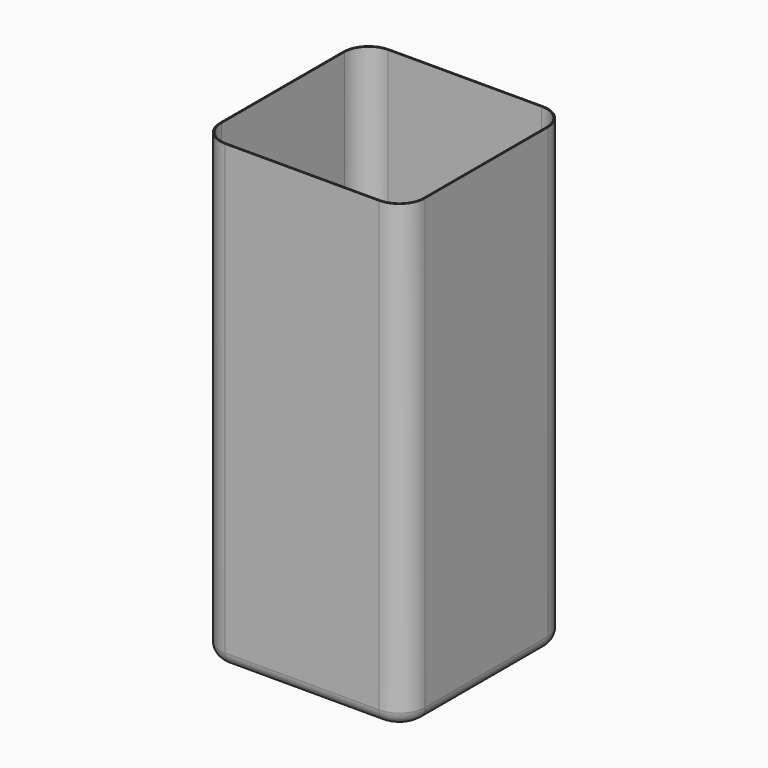
from build123d import *

# Parameters (mm, degrees)
F1_DEPTH     = 914.4
F2_R         = 25.4
F3_T1_DEPTH  = 1041.4
F3_T4_ANGLE  = 90
F3_T6_ANGLE  = 90
F3_T8_ANGLE  = 90
F3_T10_ANGLE = 90
F4_T         = -2.54


# Not quite as in the source:
# - a fillet or chamfer that OpenCascade refuses, or shapes differently, is made with other operations: its cross-section is extruded or revolved along the edge and cut away or added


with BuildPart() as f1:
    # F0 (on Top) → F1 (new body)
    with BuildSketch(Plane.XY):
        Polygon((203.2, -203.2), (203.2, 0), (203.2, 203.2), (-203.2, 203.2), (-203.2, -203.2), align=None)
    extrude(amount=F1_DEPTH)

    # F2
    f2_edges = [f1.edges().sort_by_distance(p)[0] for p in [
        (-203.2, 0, 0),
        (0, 203.2, 0),
        (0, -203.2, 0),
        (203.2, 0, 0),
    ]]
    fillet(f2_edges, radius=F2_R)

    # F3: fillet of radius 50.8 on 4 edges, made by hand

    # F3_s2 → F3_t1 (cut)
    with BuildSketch(Plane.XY):
        with BuildLine():
            ThreePointArc((-152.4, 203.2), (-188.3210244843, 188.3210244843), (-203.2, 152.4))
            Line((-203.2, 152.4), (-203.2, 203.2))
            Line((-203.2, 203.2), (-152.4, 203.2))
        make_face()
        with BuildLine():
            ThreePointArc((-152.4, -203.2), (-188.3210244843, -188.3210244843), (-203.2, -152.4))
            Line((-203.2, -152.4), (-203.2, -203.2))
            Line((-203.2, -203.2), (-152.4, -203.2))
        make_face()
        with BuildLine():
            ThreePointArc((203.2, 152.4), (188.3210244843, 188.3210244843), (152.4, 203.2))
            Line((152.4, 203.2), (203.2, 203.2))
            Line((203.2, 203.2), (203.2, 152.4))
        make_face()
        with BuildLine():
            ThreePointArc((203.2, -152.4), (188.3210244843, -188.3210244843), (152.4, -203.2))
            Line((152.4, -203.2), (203.2, -203.2))
            Line((203.2, -203.2), (203.2, -152.4))
        make_face()
    extrude(amount=F3_T1_DEPTH, mode=Mode.SUBTRACT)

    # F3_s3 → F3_t4 (revolve, cut)
    with BuildSketch(Plane.XZ.offset(152.4)):
        with BuildLine():
            ThreePointArc((177.8, 0), (195.7605122421, 7.4394877579), (203.2, 25.4))
            Line((203.2, 25.4), (203.2, 0))
            Line((203.2, 0), (177.8, 0))
        make_face()
    revolve(axis=Axis((152.4, -152.4, 0), (0, 0, -1)), revolution_arc=F3_T4_ANGLE, mode=Mode.SUBTRACT)

    # F3_s5 → F3_t6 (revolve, cut)
    with BuildSketch(Plane.YZ.offset(152.4)):
        with BuildLine():
            ThreePointArc((177.8, 0), (195.7605122421, 7.4394877579), (203.2, 25.4))
            Line((203.2, 25.4), (203.2, 0))
            Line((203.2, 0), (177.8, 0))
        make_face()
    revolve(axis=Axis((152.4, 152.4, 0), (0, 0, -1)), revolution_arc=F3_T6_ANGLE, mode=Mode.SUBTRACT)

    # F3_s7 → F3_t8 (revolve, cut)
    with BuildSketch(Plane.YZ.offset(-152.4)):
        with BuildLine():
            ThreePointArc((-177.8, 0), (-195.7605122421, 7.4394877579), (-203.2, 25.4))
            Line((-203.2, 25.4), (-203.2, 0))
            Line((-203.2, 0), (-177.8, 0))
        make_face()
    revolve(axis=Axis((-152.4, -152.4, 0), (0, 0, -1)), revolution_arc=F3_T8_ANGLE, mode=Mode.SUBTRACT)

    # F3_s9 → F3_t10 (revolve, cut)
    with BuildSketch(Plane.XZ.offset(-152.4)):
        with BuildLine():
            ThreePointArc((-177.8, 0), (-195.7605122421, 7.4394877579), (-203.2, 25.4))
            Line((-203.2, 25.4), (-203.2, 0))
            Line((-203.2, 0), (-177.8, 0))
        make_face()
    revolve(axis=Axis((-152.4, 152.4, 0), (0, 0, -1)), revolution_arc=F3_T10_ANGLE, mode=Mode.SUBTRACT)

    # F4
    f4_openings = [f1.faces().sort_by_distance(p)[0] for p in [
        (0, 0, 914.4),
    ]]
    offset(amount=F4_T, openings=f4_openings)


solid = f1.part
